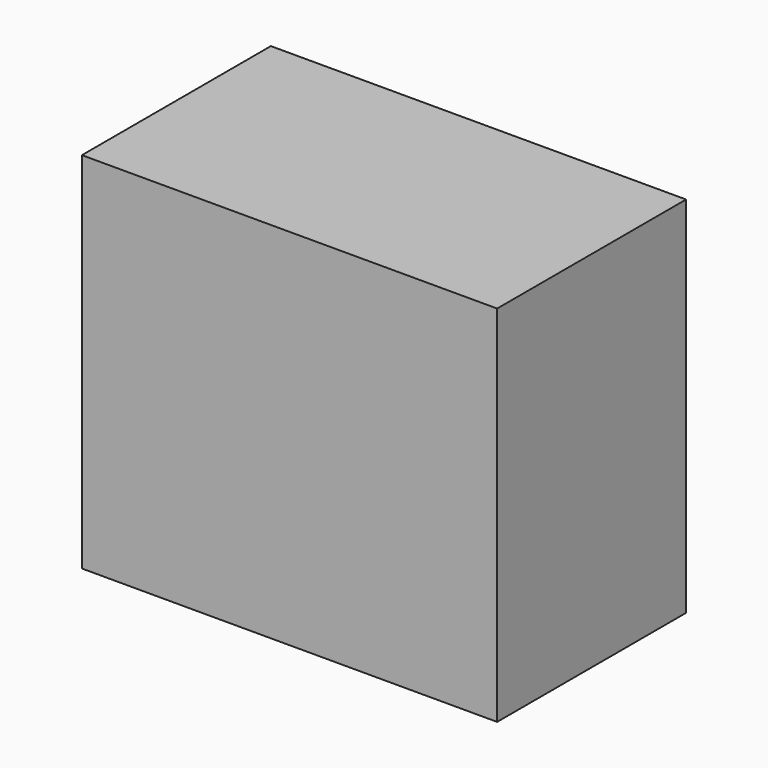
from build123d import *

# Parameters (mm, degrees)
F0_W     = 44.6580164135
F0_H     = 39.1384875402
F1_DEPTH = 25.4


# Not quite as in the source:
# - the program builds the solid bodies; features that only make, move or delete a surface that nothing else refers to are left out


with BuildPart() as f1:
    # F0 (on Front) → F1 (new body)
    with BuildSketch(Plane.XZ):
        with Locations((-82.5420636684, 34.6225094981)):
            Rectangle(F0_W, F0_H)
    extrude(amount=F1_DEPTH)


solid = f1.part
